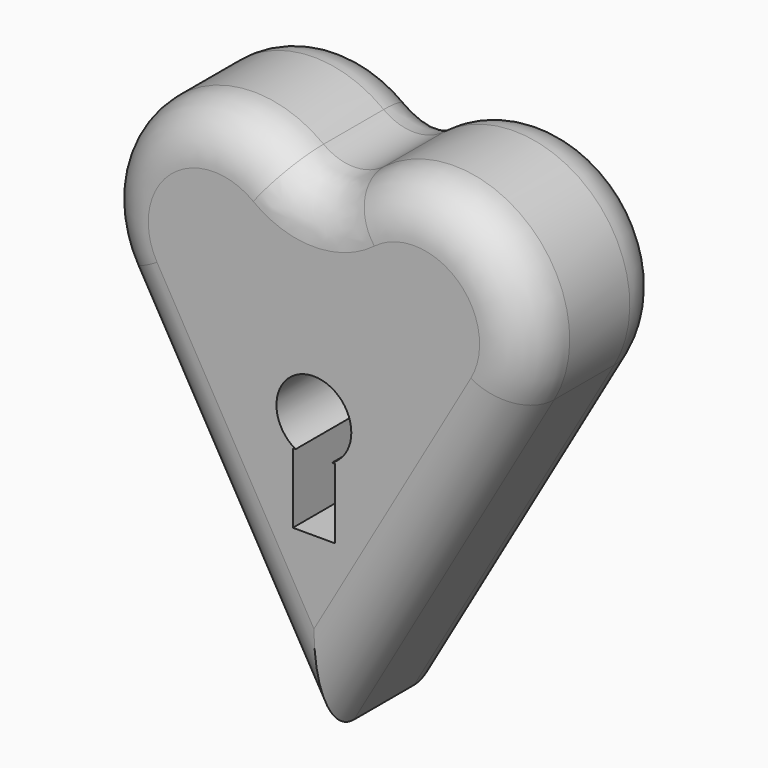
from build123d import *

# Parameters (mm, degrees)
F1_DEPTH = 35
F2_F1_R  = 10
F2_F2_R  = 10


with BuildPart() as f1:
    # F0 (on Front) → F1 (new body)
    with BuildSketch(Plane.XZ):
        with BuildLine():
            ThreePointArc((-0.0047558207, 48.9411353783), (-31.5398699376, 57.380504031), (-39.9857325354, 25.8471285283))
            Line((-39.9857325354, 25.8471285283), (0.0142674646, -43.4349037745))
            Line((0.0142674646, -43.4349037745), (40.0142674646, 25.8471285283))
            ThreePointArc((40.0142674646, 25.8471285283), (31.5541374022, 57.4077646413), (-0.0047558207, 48.9411353783))
        make_face()
        with BuildLine():
            ThreePointArc((-3.643705829, 6.997927092), (-3.7871096163, 19.9786310917), (7.4790206276, 13.5293249041))
            ThreePointArc((7.4790206276, 13.5293249041), (6.4493061876, 9.7422152878), (3.643705829, 6.997927092))
            Line((3.643705829, 6.997927092), (4.1987560689, 6.997927092))
            Line((4.1987560689, 6.997927092), (4.1987560689, -6.997927092))
            Line((4.1987560689, -6.997927092), (-4.1987560689, -6.997927092))
            Line((-4.1987560689, -6.997927092), (-4.1987560689, 6.997927092))
            Line((-4.1987560689, 6.997927092), (-3.643705829, 6.997927092))
        make_face(mode=Mode.SUBTRACT)
        with BuildLine():
            ThreePointArc((0, 25.8471285283), (-3.0951138699, 37.3934950566), (-0.0047558207, 48.9411353783))
            ThreePointArc((-0.0047558207, 48.9411353783), (3.0929066858, 37.3947693749), (0, 25.8471285283))
        make_face(mode=Mode.SUBTRACT)
        with BuildLine():
            ThreePointArc((0, 25.8471285283), (3.0929066858, 37.3947693749), (-0.0047558207, 48.9411353783))
            ThreePointArc((-0.0047558207, 48.9411353783), (-3.0951138699, 37.3934950566), (0, 25.8471285283))
        make_face()
    extrude(amount=F1_DEPTH)

    # F2: fillet of radius 10 on 4 edges, made by hand

    # F2_f1
    f2_f1_edges = [f1.edges().sort_by_distance(p)[0] for p in [
        (-0.0047558207, -17.5, 48.9411353783),
    ]]
    fillet(f2_f1_edges, radius=F2_F1_R)

    # F2_f2
    f2_f2_edges = [f1.edges().sort_by_distance(p)[0] for p in [
        (-35.2672128577, 0, 54.7003379421),
        (-35.2672128577, -35, 54.7003379421),
        (-19.9857325354, -35, -8.7938876231),
        (-19.9857325354, 0, -8.7938876231),
        (-0.0065856085, -35, 53.761031934),
        (-0.0065856085, 0, 53.761031934),
    ]]
    fillet(f2_f2_edges, radius=F2_F2_R)


solid = f1.part
